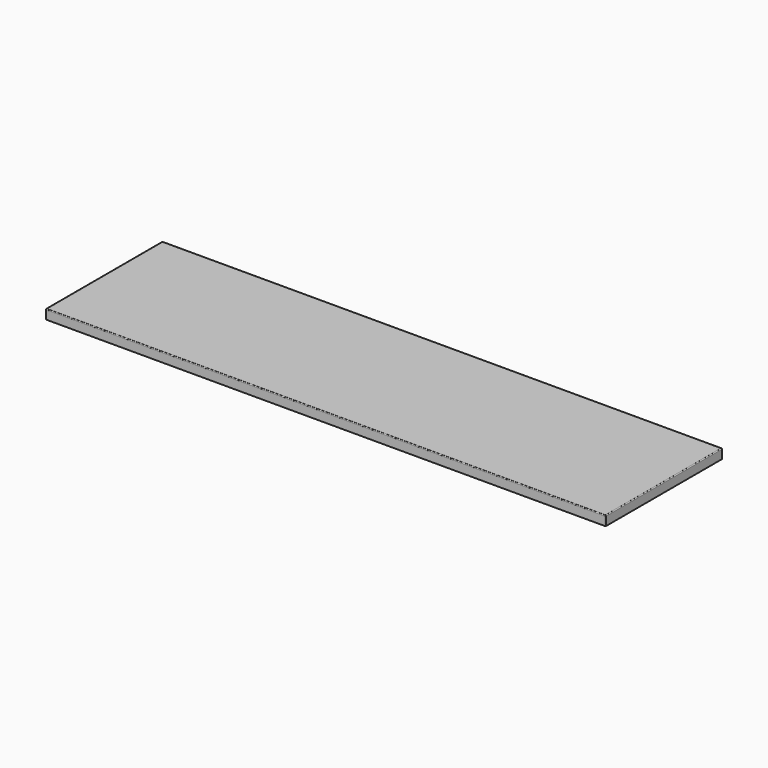
from build123d import *

# Parameters (mm, degrees)
F0_W        = 1420
F0_H        = 370
F1_DEPTH    = 24
F2_R        = 2
F3_R        = 2
F4_T1_DEPTH = 27
F4_S5_W     = 2
F4_S5_H     = 2
F4_T6_DEPTH = 2
F5_T1_DEPTH = 27
F5_S5_W     = 2
F5_S5_H     = 2
F5_T6_DEPTH = 2


# Not quite as in the source:
# - a fillet or chamfer that OpenCascade refuses, or shapes differently, is made with other operations: its cross-section is extruded or revolved along the edge and cut away or added


with BuildPart() as f1:
    # F0 (on Top) → F1 (new body)
    with BuildSketch(Plane.XY):
        with Locations((20.329669588, 0)):
            Rectangle(F0_W, F0_H)
    extrude(amount=F1_DEPTH)

    # F2
    f2_edges = [f1.edges().sort_by_distance(p)[0] for p in [
        (20.32967, -185, 24),
    ]]
    fillet(f2_edges, radius=F2_R)

    # F3
    f3_edges = [f1.edges().sort_by_distance(p)[0] for p in [
        (-689.67033, 1, 24),
        (730.32967, 1, 24),
        (20.32967, 185, 24),
    ]]
    fillet(f3_edges, radius=F3_R)

    # F4: fillet of radius 2 on 1 edges, made by hand

    # F4_s2 → F4_t1 (cut)
    with BuildSketch(Plane.XY.offset(-5)):
        with BuildLine():
            ThreePointArc((728.329669588, 185), (729.7438831503, 184.4142135624), (730.329669588, 183))
            Line((730.329669588, 183), (730.329669588, 185))
            Line((730.329669588, 185), (728.329669588, 185))
        make_face()
    extrude(amount=F4_T1_DEPTH, mode=Mode.SUBTRACT)


with BuildPart() as f4_tool4:
    # F4_s5 → F4_t6 (new body)
    with BuildSketch(Plane.XZ.offset(-183)):
        with Locations((729.329669588, 23)):
            Rectangle(F4_S5_W, F4_S5_H)
    extrude(amount=-F4_T6_DEPTH)

    # F4_s7 → F4_t8 (revolve, cut)
    with BuildSketch(Plane(origin=(728.329669588, 183, 22), x_dir=(-0.7071067812, 0, -0.7071067812), z_dir=(0.7071067812, 0, -0.7071067812))):
        with BuildLine():
            ThreePointArc((0, -2), (2, 0), (0, 2))
            Line((0, 2), (0, -2))
        make_face()
    revolve(axis=Axis((728.329669588, 183, 22), (0, 1, 0)), mode=Mode.SUBTRACT)


with BuildPart() as f1_1:
    add(f1.part)

    # F4_t3: cut F4_tool4
    add(f4_tool4.part, mode=Mode.SUBTRACT)

    # F5: fillet of radius 2 on 1 edges, made by hand

    # F5_s2 → F5_t1 (cut)
    with BuildSketch(Plane.XY.offset(-5)):
        with BuildLine():
            ThreePointArc((-689.670330412, 183), (-689.0845439744, 184.4142135624), (-687.670330412, 185))
            Line((-687.670330412, 185), (-689.670330412, 185))
            Line((-689.670330412, 185), (-689.670330412, 183))
        make_face()
    extrude(amount=F5_T1_DEPTH, mode=Mode.SUBTRACT)


with BuildPart() as f5_tool4:
    # F5_s5 → F5_t6 (new body)
    with BuildSketch(Plane.YZ.offset(-687.670330412)):
        with Locations((184, 23)):
            Rectangle(F5_S5_W, F5_S5_H)
    extrude(amount=-F5_T6_DEPTH)

    # F5_s7 → F5_t8 (revolve, cut)
    with BuildSketch(Plane(origin=(-687.670330412, 183, 22), x_dir=(0, -0.7071067812, -0.7071067812), z_dir=(0, 0.7071067812, -0.7071067812))):
        with BuildLine():
            ThreePointArc((0, -2), (2, 0), (0, 2))
            Line((0, 2), (0, -2))
        make_face()
    revolve(axis=Axis((-687.670330412, 183, 22), (-1, 0, 0)), mode=Mode.SUBTRACT)


with BuildPart() as f1_2:
    add(f1_1.part)

    # F5_t3: cut F5_tool4
    add(f5_tool4.part, mode=Mode.SUBTRACT)


solid = f1_2.part
